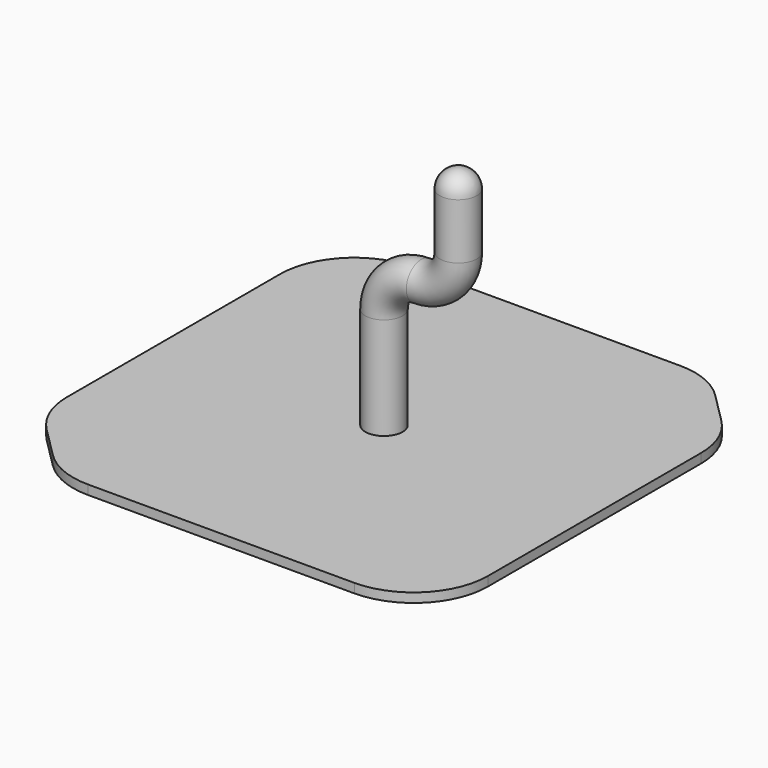
from build123d import *

# Parameters (mm, degrees)
F3_R     = 6.35
F7_W     = 152.4
F7_H     = 152.4
F8_DEPTH = 3.175
F9_DEPTH = 9.525
F10_R    = 25.4
F11_SIZE = 25.4
F12_R    = 25.4
F13_R    = 6.35


# Not quite as in the source:
# - the program builds the solid bodies; features that only make, move or delete a surface that nothing else refers to are left out


with BuildPart() as f5:
    # F5: sweep along a path in F4
    with BuildLine(Plane.XZ) as f5_path:
        Line((0, 0), (0, 25.4))
        ThreePointArc((0, 25.4), (3.7197438789, 34.3802561211), (12.7, 38.1))
        ThreePointArc((12.7, 38.1), (21.6802561211, 41.8197438789), (25.4, 50.8))
        Line((25.4, 50.8), (25.4, 76.2))
    # F3 (on Top) → F5 (sweep)
    with BuildSketch(Plane.XY):
        Circle(F3_R)
    sweep(path=f5_path.line)

    # F9 (add): a face of the model
    f9_faces = [f5.faces().sort_by_distance(p)[0] for p in [
        (0, 0, 0),
    ]]
    extrude(f9_faces, amount=F9_DEPTH)

    # F13
    f13_edges = [f5.edges().sort_by_distance(p)[0] for p in [
        (19.05, 0, 76.2),
    ]]
    fillet(f13_edges, radius=F13_R)


with BuildPart() as f8:
    # F7 (on offset) → F8 (new body)
    with BuildSketch(Plane.XY.offset(-9.525)):
        Rectangle(F7_W, F7_H)
    extrude(amount=-F8_DEPTH)

    # F10
    f10_edges = [f8.edges().sort_by_distance(p)[0] for p in [
        (76.2, -76.2, -11.1125),
        (-76.2, 76.2, -11.1125),
    ]]
    fillet(f10_edges, radius=F10_R)

    # F11
    f11_edges = [f8.edges().sort_by_distance(p)[0] for p in [
        (-76.2, -76.2, -11.1125),
        (76.2, 76.2, -11.1125),
    ]]
    chamfer(f11_edges, length=F11_SIZE)

    # F12
    f12_edges = [f8.edges().sort_by_distance(p)[0] for p in [
        (-76.2, -50.8, -11.1125),
        (-50.8, -76.2, -11.1125),
        (76.2, 50.8, -11.1125),
        (50.8, 76.2, -11.1125),
    ]]
    fillet(f12_edges, radius=F12_R)


solid = Compound([f5.part, f8.part])
